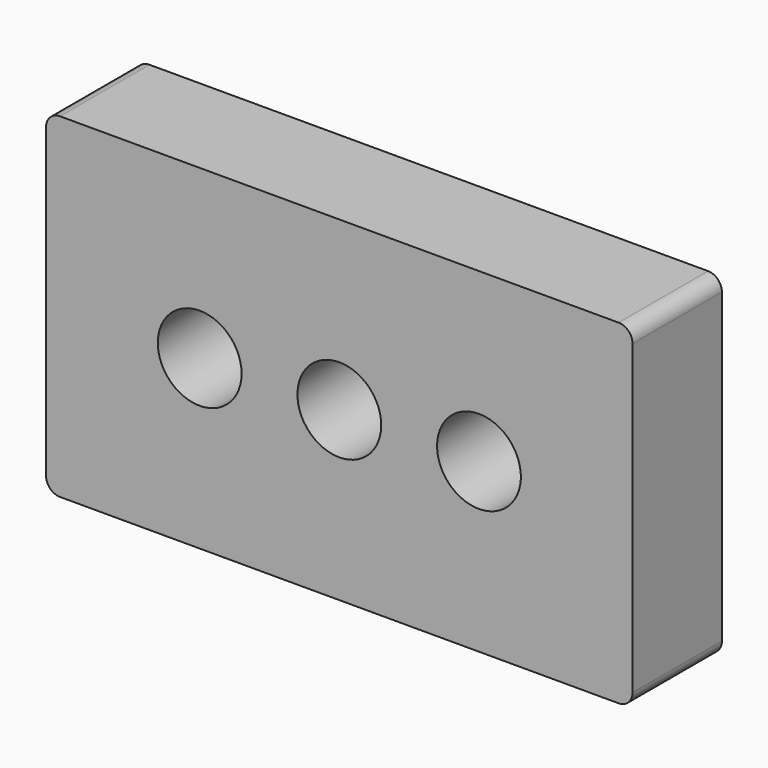
from build123d import *

# Parameters (mm, degrees)
F0_W     = 266.7
F0_H     = 152.4
F1_DEPTH = 50.8
F2_R     = 19.05
F3_DEPTH = 76.2
F4_R     = 6.35


with BuildPart() as f1:
    # F0 (on Front) → F1 (new body)
    with BuildSketch(Plane.XZ):
        Rectangle(F0_W, F0_H)
    extrude(amount=F1_DEPTH)

    # F2 (on face) → F3 (cut)
    with BuildSketch(Plane.XZ.offset(50.8)):
        with BuildLine():
            ThreePointArc((-19.05, 0), (0, -19.05), (19.05, 0))
            ThreePointArc((19.05, 0), (0, 19.05), (-19.05, 0))
        make_face()
        with Locations((-63.5, 0)):
            Circle(F2_R)
        with BuildLine():
            ThreePointArc((82.55, 0), (63.5, 19.05), (44.45, 0))
            ThreePointArc((44.45, 0), (63.5, -19.05), (82.55, 0))
        make_face()
    extrude(amount=-F3_DEPTH, mode=Mode.SUBTRACT)

    # F4
    f4_edges = [f1.edges().sort_by_distance(p)[0] for p in [
        (133.35, -25.4, 76.2),
        (133.35, -25.4, -76.2),
        (-133.35, -25.4, 76.2),
        (-133.35, -25.4, -76.2),
    ]]
    fillet(f4_edges, radius=F4_R)


solid = f1.part
